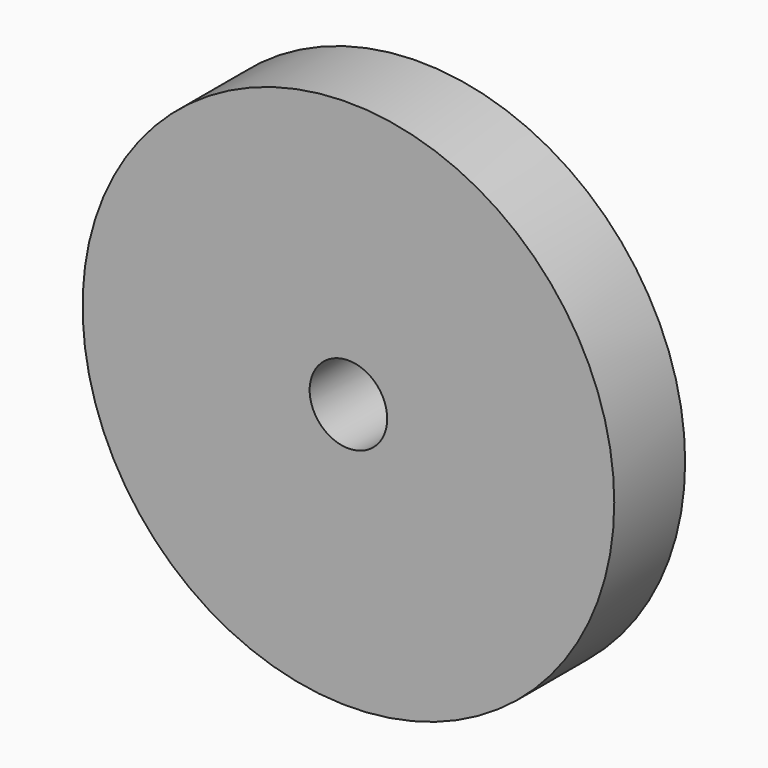
from build123d import *

# Parameters (mm, degrees)
F2_R     = 12
F2_R_2   = 1.75
F3_DEPTH = 4


# Not quite as in the source:
# - the program builds the solid bodies; features that only make, move or delete a surface that nothing else refers to are left out


with BuildPart() as f3:
    # F2 (on Front) → F3 (new body)
    with BuildSketch(Plane.XZ):
        Circle(F2_R)
        Circle(F2_R_2, mode=Mode.SUBTRACT)
    extrude(amount=F3_DEPTH)


solid = f3.part
